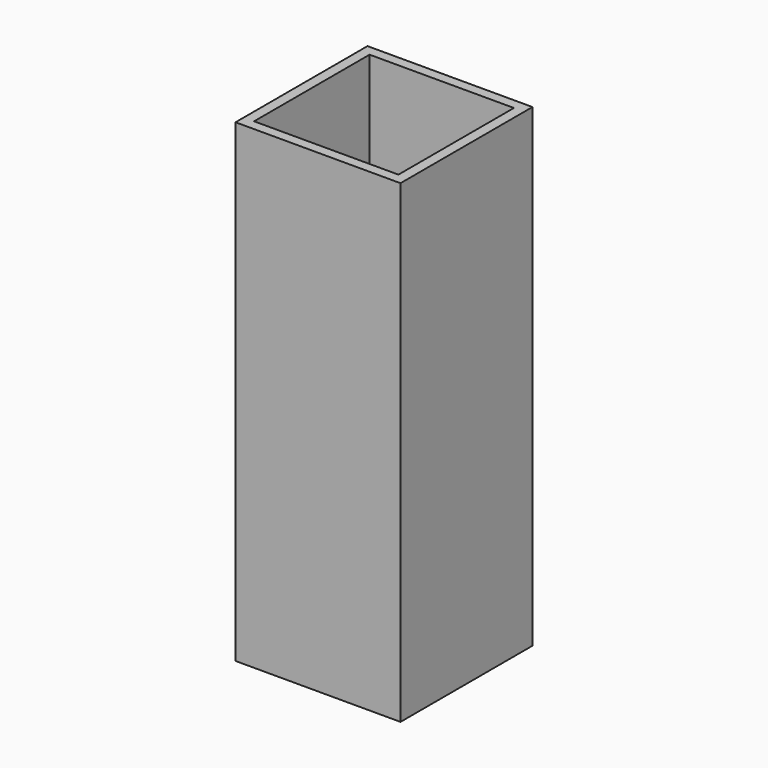
from build123d import *

# Parameters (mm, degrees)
F1_W     = 25.4
F1_H     = 25.4
F2_DEPTH = 73.025
F3_T     = -1.5875
F4_DEPTH = 1.5885


# Not quite as in the source:
# - a variable given as a bare number and used for a length is read in inches; the dataset says mm whatever the document's units were


with BuildPart() as f2:
    # F1 (on Top) → F2 (new body)
    with BuildSketch(Plane.XY):
        Rectangle(F1_W, F1_H)
    extrude(amount=F2_DEPTH)

    # F3
    f3_openings = [f2.faces().sort_by_distance(p)[0] for p in [
        (0, 0, 73.025),
    ]]
    offset(amount=F3_T, openings=f3_openings)

    # F4 (cut, through all): a face of the model
    f4_faces = [f2.faces().sort_by_distance(p)[0] for p in [
        (0, 0, 1.5875),
    ]]
    extrude(f4_faces, amount=-F4_DEPTH, mode=Mode.SUBTRACT)


solid = f2.part
